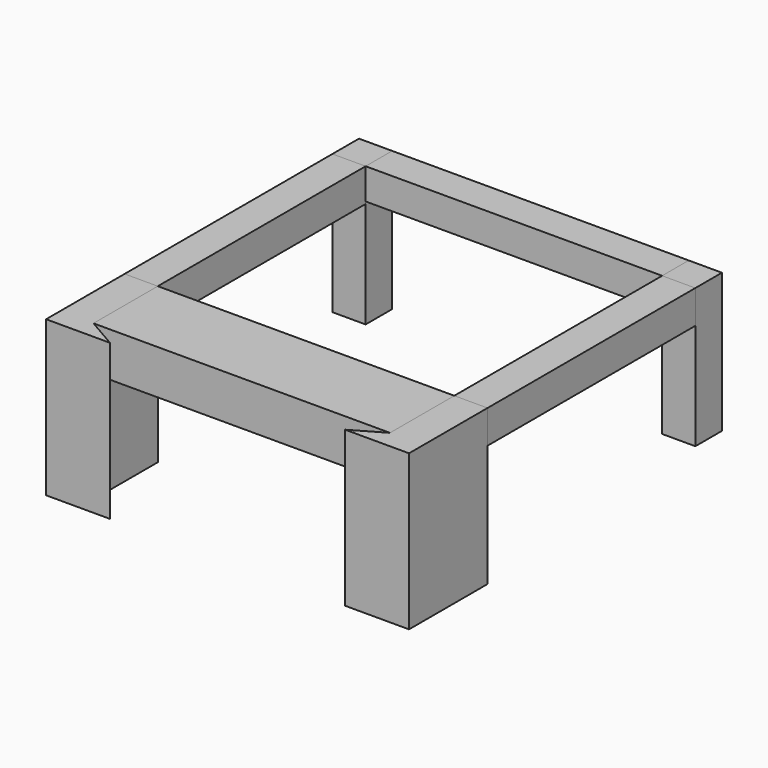
from build123d import *

# Parameters (mm, degrees)
F0_W     = 3.81
F0_H     = 9.2202
F1_DEPTH = 17.78
F2_DEPTH = 3.81
F0_H_2   = 3.81
F3_DEPTH = 15.9766
F0_W_2   = 34.0106
F4_DEPTH = 5.08
F5_DEPTH = 3.556


# Not quite as in the source:
# - a feature names something its author has since deleted; it is built from what else it names


with BuildPart() as f1:
    # F0 (on Top) → F1 (new body)
    with BuildSketch(Plane.XY):
        with Locations((-21.3418023896, -4.6101)):
            Rectangle(F0_W, F0_H)
        Polygon((-15.9172751486, -11.2522), (-19.4368023896, -9.2202), (-23.2468023896, -9.2202), (-23.2468023896, -11.2522), align=None)
    extrude(amount=-F1_DEPTH)


with BuildPart() as f1b:
    # F0 (on Top) → F1, piece 2 (new body)
    with BuildSketch(Plane.XY):
        Polygon((18.3837976104, -9.2202), (14.5737976104, -9.2202), (11.0542703694, -11.2522), (18.3837976104, -11.2522), align=None)
        with Locations((16.4787976104, -4.6101)):
            Rectangle(F0_W, F0_H)
    extrude(amount=-F1_DEPTH)


with BuildPart() as f2:
    # F0 (on Top) → F2 (new body)
    with BuildSketch(Plane.XY):
        Polygon((-23.2468023896, 0), (-19.4368023896, 0), (-19.4368023896, 26.035), (-19.4368023896, 29.799785465), (-23.2468023896, 29.799785465), (-23.2468023896, 26.035), align=None)
    extrude(amount=-F2_DEPTH)


with BuildPart() as f2b:
    # F0 (on Top) → F2, piece 2 (new body)
    with BuildSketch(Plane.XY):
        Polygon((14.5737976104, 26.035), (14.5737976104, 0), (18.3837976104, 0), (18.3837976104, 26.035), (18.3837976104, 29.799785465), (14.5737976104, 29.799785465), align=None)
    extrude(amount=-F2_DEPTH)


with BuildPart() as f3:
    # F0 (on Top) → F3 (new body)
    with BuildSketch(Plane.XY):
        with Locations((-21.3418023896, 31.704785465)):
            Rectangle(F0_W, F0_H_2)
    extrude(amount=-F3_DEPTH)


with BuildPart() as f3b:
    # F0 (on Top) → F3, piece 2 (new body)
    with BuildSketch(Plane.XY):
        with Locations((16.4787976104, 31.704785465)):
            Rectangle(F0_W, F0_H_2)
    extrude(amount=-F3_DEPTH)


with BuildPart() as f4:
    # F0 (on Top) → F4 (new body)
    with BuildSketch(Plane.XY):
        with Locations((-2.4315023896, -4.6101)):
            Rectangle(F0_W_2, F0_H)
    extrude(amount=-F4_DEPTH)


with BuildPart() as f5:
    # F0 (on Top) → F5 (new body)
    with BuildSketch(Plane.XY):
        with Locations((-2.4315023896, 31.704785465)):
            Rectangle(F0_W_2, F0_H_2)
    extrude(amount=-F5_DEPTH)


solid = Compound([f1.part, f1b.part, f2.part, f2b.part, f3.part, f3b.part, f4.part, f5.part])
